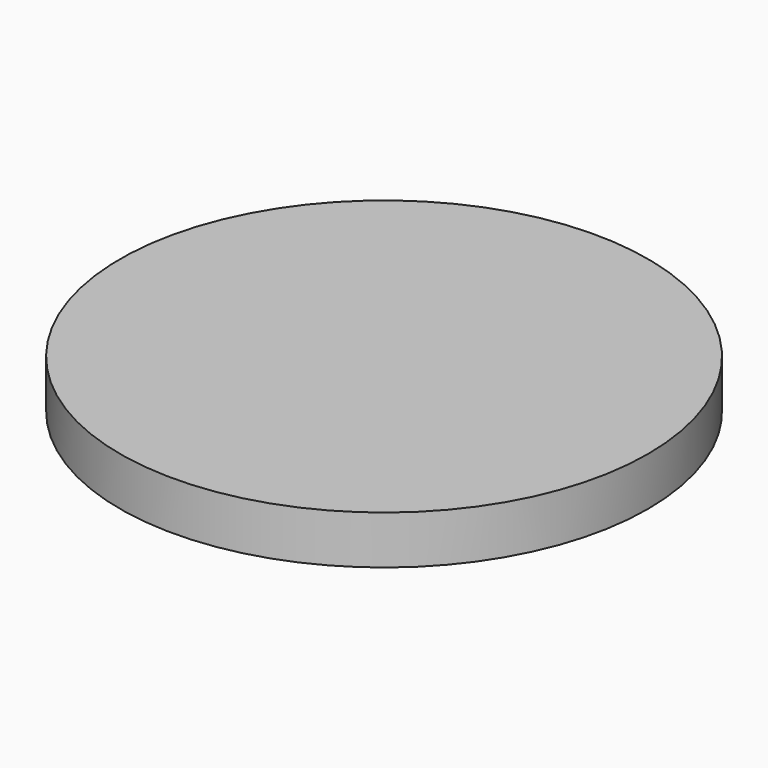
from build123d import *

# Parameters (mm, degrees)
F0_R     = 120
F1_DEPTH = 22


# Not quite as in the source:
# - a feature names something its author has since deleted; it is built from what else it names


with BuildPart() as f1:
    # F0 (on Top) → F1 (new body)
    with BuildSketch(Plane.XY):
        Circle(F0_R)
    extrude(amount=-F1_DEPTH)


solid = f1.part
